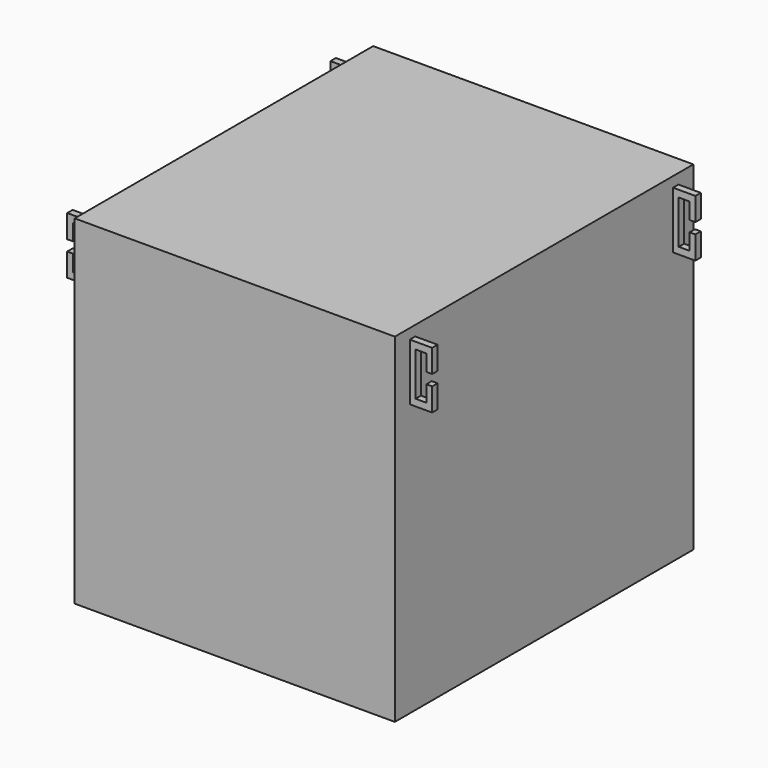
from build123d import *

# Parameters (mm, degrees)
F0_W             = 944
F0_H             = 1000
F1_DEPTH         = 550
F4_DEPTH         = 10
F4_COPIES2_COUNT = 2


# Not quite as in the source:
# - a pattern or mirror of a feature is missing from the dataset's text; its kind, count and spacing are read off the source's solid


with BuildPart() as f1:
    # F0 (on Front) → F1 (new body, symmetric)
    with BuildSketch(Plane.XZ):
        Rectangle(F0_W, F0_H)
    extrude(amount=F1_DEPTH, both=True)

    # F3 (on offset) → F4 (join, symmetric)
    with BuildSketch(Plane.XZ.offset(485)):
        Polygon((538, 470), (472, 470), (472, 302), (538, 302), (538, 370), (521, 370), (521, 322), (489, 322), (489, 450), (521, 450), (521, 402), (538, 402), align=None)
    f4 = extrude(amount=F4_DEPTH, both=True)

    # F4_copies: F4 across plane
    add(f4.mirror(Plane.ZX))

    # F4_copies1: F4 across plane
    add(f4.mirror(Plane(origin=(0, 0, 0), x_dir=(0, 0, -1), z_dir=(-1, 0, 0))))

    # F4_copies2: F4 ×2 about axis
    f4_copies2_axis = Axis((0, 0, 0), (0, 0, 1))
    for i in range(1, F4_COPIES2_COUNT):
        add(f4.rotate(f4_copies2_axis, i * 360 / F4_COPIES2_COUNT))


solid = f1.part
